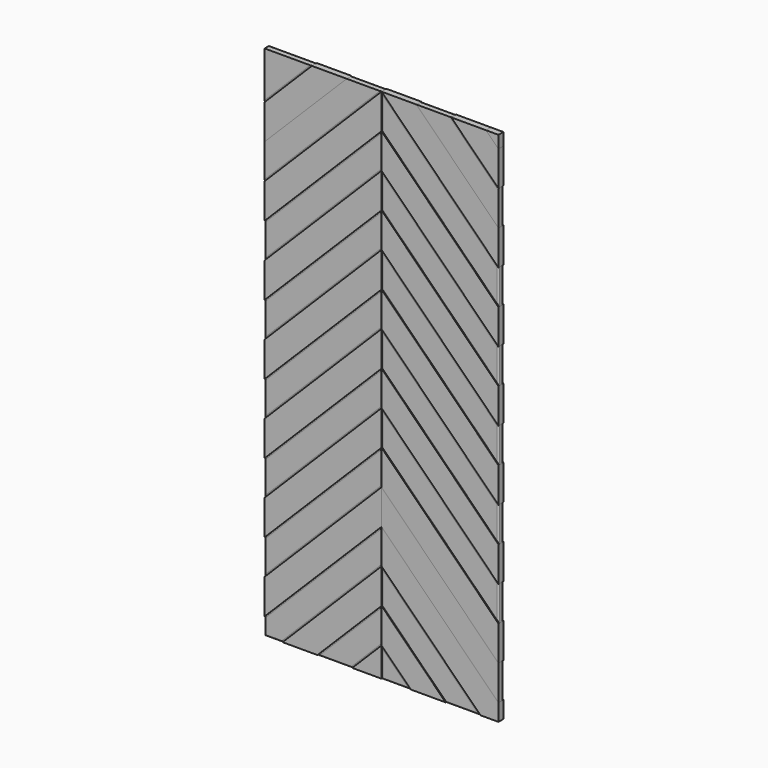
from build123d import *

# Parameters (mm, degrees)
F1_DEPTH = 25.4
F2_R     = 5.08
F2_2_R   = 5.08
F2_3_R   = 5.08
F2_4_R   = 5.08
F2_5_R   = 5.08
F2_6_R   = 5.08
F2_7_R   = 5.08
F2_8_R   = 5.08
F2_9_R   = 5.08
F2_10_R  = 5.08
F2_11_R  = 5.08
F2_12_R  = 5.08
F2_13_R  = 5.08
F2_14_R  = 5.08
F2_15_R  = 5.08
F2_16_R  = 5.08
F2_17_R  = 5.08
F2_18_R  = 5.08
F3_DEPTH = 25.4


with BuildPart() as f1:
    # F0 (on Front) → F1 (new body)
    with BuildSketch(Plane.XZ):
        Polygon((-482.6, 1015.492), (-431.292, 1066.8), (-482.6, 1066.8), align=None)
        Polygon((-482.6, 871.728), (-287.528, 1066.8), (-431.292, 1066.8), (-482.6, 1015.492), align=None)
    extrude(amount=F1_DEPTH)

    # F2
    f2_edges = [f1.edges().sort_by_distance(p)[0] for p in [
        (-385.064, -25.4, 969.264),
        (-482.6, 0, 969.264),
        (-385.064, 0, 969.264),
        (-385.064, 0, 1066.8),
    ]]
    fillet(f2_edges, radius=F2_R)


with BuildPart() as f1b:
    # F0 (on Front) → F1, piece 2 (new body)
    with BuildSketch(Plane.XZ):
        Polygon((431.292, 1066.8), (482.6, 1015.492), (482.6, 1066.8), align=None)
    extrude(amount=F1_DEPTH)


with BuildPart() as f1c:
    # F0 (on Front) → F1, piece 3 (new body)
    with BuildSketch(Plane.XZ):
        Polygon((0, -1066.8), (120.904, -1066.8), (0, -945.896), align=None)
    extrude(amount=F1_DEPTH)

    # F2#17
    f2_17_edges = [f1c.edges().sort_by_distance(p)[0] for p in [
        (60.452, -25.4, -1066.8),
        (60.452, -25.4, -1006.348),
        (0, -25.4, -1006.348),
        (60.452, 0, -1066.8),
        (60.452, 0, -1006.348),
        (0, 0, -1006.348),
    ]]
    fillet(f2_17_edges, radius=F2_17_R)


with BuildPart() as f1d:
    # F0 (on Front) → F1, piece 4 (new body)
    with BuildSketch(Plane.XZ):
        Polygon((0, -945.896), (0, -802.132), (-264.668, -1066.8), (-120.904, -1066.8), align=None)
    extrude(amount=F1_DEPTH)

    # F2#15
    f2_15_edges = [f1d.edges().sort_by_distance(p)[0] for p in [
        (-132.334, -25.4, -934.466),
        (-192.786, -25.4, -1066.8),
        (-60.452, -25.4, -1006.348),
        (0, -25.4, -874.014),
        (-132.334, 0, -934.466),
        (-192.786, 0, -1066.8),
        (-60.452, 0, -1006.348),
        (0, 0, -874.014),
    ]]
    fillet(f2_15_edges, radius=F2_15_R)


with BuildPart() as f1e:
    # F0 (on Front) → F1, piece 5 (new body)
    with BuildSketch(Plane.XZ):
        Polygon((264.668, -1066.8), (408.432, -1066.8), (0, -658.368), (0, -802.132), align=None)
    extrude(amount=F1_DEPTH)

    # F2#16
    f2_16_edges = [f1e.edges().sort_by_distance(p)[0] for p in [
        (132.334, -25.4, -934.466),
        (336.55, -25.4, -1066.8),
        (204.216, -25.4, -862.584),
        (0, -25.4, -730.25),
        (132.334, 0, -934.466),
        (336.55, 0, -1066.8),
        (204.216, 0, -862.584),
        (0, 0, -730.25),
    ]]
    fillet(f2_16_edges, radius=F2_16_R)


with BuildPart() as f1f:
    # F0 (on Front) → F1, piece 6 (new body)
    with BuildSketch(Plane.XZ):
        Polygon((-408.432, -1066.8), (0, -658.368), (0, -514.604), (-482.6, -997.204), (-482.6, -1066.8), align=None)
    extrude(amount=F1_DEPTH)

    # F2#14
    f2_14_edges = [f1f.edges().sort_by_distance(p)[0] for p in [
        (-204.216, -25.4, -862.584),
        (0, -25.4, -586.486),
        (-241.3, -25.4, -755.904),
        (-482.6, -25.4, -1032.002),
        (-445.516, -25.4, -1066.8),
        (-204.216, 0, -862.584),
        (0, 0, -586.486),
        (-241.3, 0, -755.904),
        (-482.6, 0, -1032.002),
        (-445.516, 0, -1066.8),
    ]]
    fillet(f2_14_edges, radius=F2_14_R)


with BuildPart() as f1g:
    # F0 (on Front) → F1, piece 7 (new body)
    with BuildSketch(Plane.XZ):
        Polygon((0, -514.604), (482.6, -997.204), (482.6, -853.44), (0, -370.84), align=None)
    extrude(amount=F1_DEPTH)

    # F2#18
    f2_18_edges = [f1g.edges().sort_by_distance(p)[0] for p in [
        (0, 0, -442.722),
        (241.3, 0, -755.904),
        (482.6, 0, -925.322),
        (241.3, 0, -612.14),
    ]]
    fillet(f2_18_edges, radius=F2_18_R)


with BuildPart() as f1h:
    # F0 (on Front) → F1, piece 8 (new body)
    with BuildSketch(Plane.XZ):
        Polygon((-482.6, -853.44), (0, -370.84), (0, -227.076), (-482.6, -709.676), align=None)
    extrude(amount=F1_DEPTH)

    # F2#13
    f2_13_edges = [f1h.edges().sort_by_distance(p)[0] for p in [
        (-241.3, -25.4, -612.14),
        (0, -25.4, -298.958),
        (-241.3, -25.4, -468.376),
        (-482.6, -25.4, -781.558),
        (-241.3, 0, -612.14),
        (0, 0, -298.958),
        (-241.3, 0, -468.376),
        (-482.6, 0, -781.558),
    ]]
    fillet(f2_13_edges, radius=F2_13_R)


with BuildPart() as f1i:
    # F0 (on Front) → F1, piece 9 (new body)
    with BuildSketch(Plane.XZ):
        Polygon((0, -227.076), (482.6, -709.676), (482.6, -565.912), (0, -83.312), align=None)
    extrude(amount=F1_DEPTH)

    # F2#12
    f2_12_edges = [f1i.edges().sort_by_distance(p)[0] for p in [
        (0, -25.4, -155.194),
        (241.3, -25.4, -468.376),
        (482.6, -25.4, -637.794),
        (241.3, -25.4, -324.612),
        (0, 0, -155.194),
        (241.3, 0, -468.376),
        (482.6, 0, -637.794),
        (241.3, 0, -324.612),
    ]]
    fillet(f2_12_edges, radius=F2_12_R)


with BuildPart() as f1j:
    # F0 (on Front) → F1, piece 10 (new body)
    with BuildSketch(Plane.XZ):
        Polygon((-482.6, -565.912), (0, -83.312), (0, 60.452), (-482.6, -422.148), align=None)
    extrude(amount=F1_DEPTH)

    # F2#11
    f2_11_edges = [f1j.edges().sort_by_distance(p)[0] for p in [
        (-482.6, -25.4, -494.03),
        (-241.3, -25.4, -324.612),
        (0, -25.4, -11.43),
        (-241.3, -25.4, -180.848),
        (-482.6, 0, -494.03),
        (-241.3, 0, -324.612),
        (0, 0, -11.43),
        (-241.3, 0, -180.848),
    ]]
    fillet(f2_11_edges, radius=F2_11_R)


with BuildPart() as f1k:
    # F0 (on Front) → F1, piece 11 (new body)
    with BuildSketch(Plane.XZ):
        Polygon((0, 60.452), (482.6, -422.148), (482.6, -278.384), (0, 204.216), align=None)
    extrude(amount=F1_DEPTH)

    # F2#9
    f2_9_edges = [f1k.edges().sort_by_distance(p)[0] for p in [
        (241.3, -25.4, -37.084),
        (0, -25.4, 132.334),
        (241.3, -25.4, -180.848),
        (482.6, -25.4, -350.266),
        (241.3, 0, -37.084),
        (0, 0, 132.334),
        (241.3, 0, -180.848),
        (482.6, 0, -350.266),
    ]]
    fillet(f2_9_edges, radius=F2_9_R)


with BuildPart() as f1l:
    # F0 (on Front) → F1, piece 12 (new body)
    with BuildSketch(Plane.XZ):
        Polygon((-482.6, -278.384), (0, 204.216), (0, 347.98), (-482.6, -134.62), align=None)
    extrude(amount=F1_DEPTH)

    # F2#10
    f2_10_edges = [f1l.edges().sort_by_distance(p)[0] for p in [
        (-241.3, -25.4, -37.084),
        (0, -25.4, 276.098),
        (-241.3, -25.4, 106.68),
        (-482.6, -25.4, -206.502),
        (-241.3, 0, -37.084),
        (0, 0, 276.098),
        (-241.3, 0, 106.68),
        (-482.6, 0, -206.502),
    ]]
    fillet(f2_10_edges, radius=F2_10_R)


with BuildPart() as f1m:
    # F0 (on Front) → F1, piece 13 (new body)
    with BuildSketch(Plane.XZ):
        Polygon((0, 347.98), (482.6, -134.62), (482.6, 9.144), (0, 491.744), align=None)
    extrude(amount=F1_DEPTH)

    # F2#8
    f2_8_edges = [f1m.edges().sort_by_distance(p)[0] for p in [
        (241.3, -25.4, 250.444),
        (0, -25.4, 419.862),
        (241.3, -25.4, 106.68),
        (482.6, -25.4, -62.738),
        (241.3, 0, 250.444),
        (0, 0, 419.862),
        (241.3, 0, 106.68),
        (482.6, 0, -62.738),
    ]]
    fillet(f2_8_edges, radius=F2_8_R)


with BuildPart() as f1n:
    # F0 (on Front) → F1, piece 14 (new body)
    with BuildSketch(Plane.XZ):
        Polygon((-482.6, 9.144), (0, 491.744), (0, 635.508), (-482.6, 152.908), align=None)
    extrude(amount=F1_DEPTH)

    # F2#7
    f2_7_edges = [f1n.edges().sort_by_distance(p)[0] for p in [
        (-241.3, -25.4, 250.444),
        (0, -25.4, 563.626),
        (-241.3, -25.4, 394.208),
        (-482.6, -25.4, 81.026),
        (-241.3, 0, 250.444),
        (0, 0, 563.626),
        (-241.3, 0, 394.208),
        (-482.6, 0, 81.026),
    ]]
    fillet(f2_7_edges, radius=F2_7_R)


with BuildPart() as f1o:
    # F0 (on Front) → F1, piece 15 (new body)
    with BuildSketch(Plane.XZ):
        Polygon((0, 635.508), (482.6, 152.908), (482.6, 296.672), (0, 779.272), align=None)
    extrude(amount=F1_DEPTH)

    # F2#5
    f2_5_edges = [f1o.edges().sort_by_distance(p)[0] for p in [
        (241.3, -25.4, 537.972),
        (0, -25.4, 707.39),
        (241.3, -25.4, 394.208),
        (482.6, -25.4, 224.79),
        (241.3, 0, 537.972),
        (0, 0, 707.39),
        (241.3, 0, 394.208),
        (482.6, 0, 224.79),
    ]]
    fillet(f2_5_edges, radius=F2_5_R)


with BuildPart() as f1p:
    # F0 (on Front) → F1, piece 16 (new body)
    with BuildSketch(Plane.XZ):
        Polygon((-482.6, 296.672), (0, 779.272), (0, 923.036), (-482.6, 440.436), align=None)
    extrude(amount=F1_DEPTH)

    # F2#6
    f2_6_edges = [f1p.edges().sort_by_distance(p)[0] for p in [
        (-241.3, -25.4, 537.972),
        (0, -25.4, 851.154),
        (-241.3, -25.4, 681.736),
        (-482.6, -25.4, 368.554),
        (-241.3, 0, 537.972),
        (0, 0, 851.154),
        (-241.3, 0, 681.736),
        (-482.6, 0, 368.554),
    ]]
    fillet(f2_6_edges, radius=F2_6_R)


with BuildPart() as f1q:
    # F0 (on Front) → F1, piece 17 (new body)
    with BuildSketch(Plane.XZ):
        Polygon((0, 923.036), (482.6, 440.436), (482.6, 584.2), (0, 1066.8), align=None)
    extrude(amount=F1_DEPTH)

    # F2#3
    f2_3_edges = [f1q.edges().sort_by_distance(p)[0] for p in [
        (0, 0, 994.918),
        (241.3, -25.4, 825.5),
        (482.6, -25.4, 512.318),
        (0, -25.4, 994.918),
        (241.3, -25.4, 681.736),
        (482.6, 0, 512.318),
        (241.3, 0, 825.5),
        (241.3, 0, 681.736),
    ]]
    fillet(f2_3_edges, radius=F2_3_R)


with BuildPart() as f1r:
    # F0 (on Front) → F1, piece 18 (new body)
    with BuildSketch(Plane.XZ):
        Polygon((-482.6, 584.2), (0, 1066.8), (-143.764, 1066.8), (-482.6, 727.964), align=None)
    extrude(amount=F1_DEPTH)

    # F2#2
    f2_2_edges = [f1r.edges().sort_by_distance(p)[0] for p in [
        (-313.182, 0, 897.382),
        (-241.3, -25.4, 825.5),
        (-482.6, 0, 656.082),
        (-241.3, 0, 825.5),
        (-71.882, 0, 1066.8),
    ]]
    fillet(f2_2_edges, radius=F2_2_R)


with BuildPart() as f1s:
    # F0 (on Front) → F1, piece 19 (new body)
    with BuildSketch(Plane.XZ):
        Polygon((143.764, 1066.8), (482.6, 727.964), (482.6, 871.728), (287.528, 1066.8), align=None)
    extrude(amount=F1_DEPTH)

    # F2#4
    f2_4_edges = [f1s.edges().sort_by_distance(p)[0] for p in [
        (385.064, -25.4, 969.264),
        (313.182, 0, 897.382),
        (385.064, 0, 969.264),
        (215.646, 0, 1066.8),
        (482.6, 0, 799.846),
    ]]
    fillet(f2_4_edges, radius=F2_4_R)


with BuildPart() as f3:
    # F0 (on Front) → F3 (new body)
    with BuildSketch(Plane.XZ):
        Polygon((-120.904, -1066.8), (0, -1066.8), (0, -945.896), align=None)
    extrude(amount=F3_DEPTH)


with BuildPart() as f3b:
    # F0 (on Front) → F3, piece 2 (new body)
    with BuildSketch(Plane.XZ):
        Polygon((0, -802.132), (0, -658.368), (-408.432, -1066.8), (-264.668, -1066.8), align=None)
    extrude(amount=F3_DEPTH)


with BuildPart() as f3c:
    # F0 (on Front) → F3, piece 3 (new body)
    with BuildSketch(Plane.XZ):
        Polygon((120.904, -1066.8), (264.668, -1066.8), (0, -802.132), (0, -945.896), align=None)
    extrude(amount=F3_DEPTH)


with BuildPart() as f3d:
    # F0 (on Front) → F3, piece 4 (new body)
    with BuildSketch(Plane.XZ):
        Polygon((408.432, -1066.8), (482.6, -1066.8), (482.6, -997.204), (0, -514.604), (0, -658.368), align=None)
    extrude(amount=F3_DEPTH)


with BuildPart() as f3e:
    # F0 (on Front) → F3, piece 5 (new body)
    with BuildSketch(Plane.XZ):
        Polygon((0, -370.84), (482.6, -853.44), (482.6, -709.676), (0, -227.076), align=None)
    extrude(amount=F3_DEPTH)


with BuildPart() as f3f:
    # F0 (on Front) → F3, piece 6 (new body)
    with BuildSketch(Plane.XZ):
        Polygon((-482.6, -997.204), (0, -514.604), (0, -370.84), (-482.6, -853.44), align=None)
    extrude(amount=F3_DEPTH)


with BuildPart() as f3g:
    # F0 (on Front) → F3, piece 7 (new body)
    with BuildSketch(Plane.XZ):
        Polygon((-482.6, -709.676), (0, -227.076), (0, -83.312), (-482.6, -565.912), align=None)
    extrude(amount=F3_DEPTH)


with BuildPart() as f3h:
    # F0 (on Front) → F3, piece 8 (new body)
    with BuildSketch(Plane.XZ):
        Polygon((-482.6, -422.148), (0, 60.452), (0, 204.216), (-482.6, -278.384), align=None)
    extrude(amount=F3_DEPTH)


with BuildPart() as f3i:
    # F0 (on Front) → F3, piece 9 (new body)
    with BuildSketch(Plane.XZ):
        Polygon((0, -83.312), (482.6, -565.912), (482.6, -422.148), (0, 60.452), align=None)
    extrude(amount=F3_DEPTH)


with BuildPart() as f3j:
    # F0 (on Front) → F3, piece 10 (new body)
    with BuildSketch(Plane.XZ):
        Polygon((0, 204.216), (482.6, -278.384), (482.6, -134.62), (0, 347.98), align=None)
    extrude(amount=F3_DEPTH)


with BuildPart() as f3k:
    # F0 (on Front) → F3, piece 11 (new body)
    with BuildSketch(Plane.XZ):
        Polygon((-482.6, -134.62), (0, 347.98), (0, 491.744), (-482.6, 9.144), align=None)
    extrude(amount=F3_DEPTH)


with BuildPart() as f3l:
    # F0 (on Front) → F3, piece 12 (new body)
    with BuildSketch(Plane.XZ):
        Polygon((0, 491.744), (482.6, 9.144), (482.6, 152.908), (0, 635.508), align=None)
    extrude(amount=F3_DEPTH)


with BuildPart() as f3m:
    # F0 (on Front) → F3, piece 13 (new body)
    with BuildSketch(Plane.XZ):
        Polygon((-482.6, 152.908), (0, 635.508), (0, 779.272), (-482.6, 296.672), align=None)
    extrude(amount=F3_DEPTH)


with BuildPart() as f3n:
    # F0 (on Front) → F3, piece 14 (new body)
    with BuildSketch(Plane.XZ):
        Polygon((-482.6, 440.436), (0, 923.036), (0, 1066.8), (-482.6, 584.2), align=None)
    extrude(amount=F3_DEPTH)


with BuildPart() as f3o:
    # F0 (on Front) → F3, piece 15 (new body)
    with BuildSketch(Plane.XZ):
        Polygon((0, 779.272), (482.6, 296.672), (482.6, 440.436), (0, 923.036), align=None)
    extrude(amount=F3_DEPTH)


with BuildPart() as f3p:
    # F0 (on Front) → F3, piece 16 (new body)
    with BuildSketch(Plane.XZ):
        Polygon((0, 1066.8), (482.6, 584.2), (482.6, 727.964), (143.764, 1066.8), align=None)
    extrude(amount=F3_DEPTH)


with BuildPart() as f3q:
    # F0 (on Front) → F3, piece 17 (new body)
    with BuildSketch(Plane.XZ):
        Polygon((-482.6, 727.964), (-143.764, 1066.8), (-287.528, 1066.8), (-482.6, 871.728), align=None)
    extrude(amount=F3_DEPTH)


with BuildPart() as f3r:
    # F0 (on Front) → F3, piece 18 (new body)
    with BuildSketch(Plane.XZ):
        Polygon((287.528, 1066.8), (482.6, 871.728), (482.6, 1015.492), (431.292, 1066.8), align=None)
    extrude(amount=F3_DEPTH)


solid = Compound([f1.part, f1b.part, f1c.part, f1d.part, f1e.part, f1f.part, f1g.part, f1h.part, f1i.part, f1j.part, f1k.part, f1l.part, f1m.part, f1n.part, f1o.part, f1p.part, f1q.part, f1r.part, f1s.part, f3.part, f3b.part, f3c.part, f3d.part, f3e.part, f3f.part, f3g.part, f3h.part, f3i.part, f3j.part, f3k.part, f3l.part, f3m.part, f3n.part, f3o.part, f3p.part, f3q.part, f3r.part])
